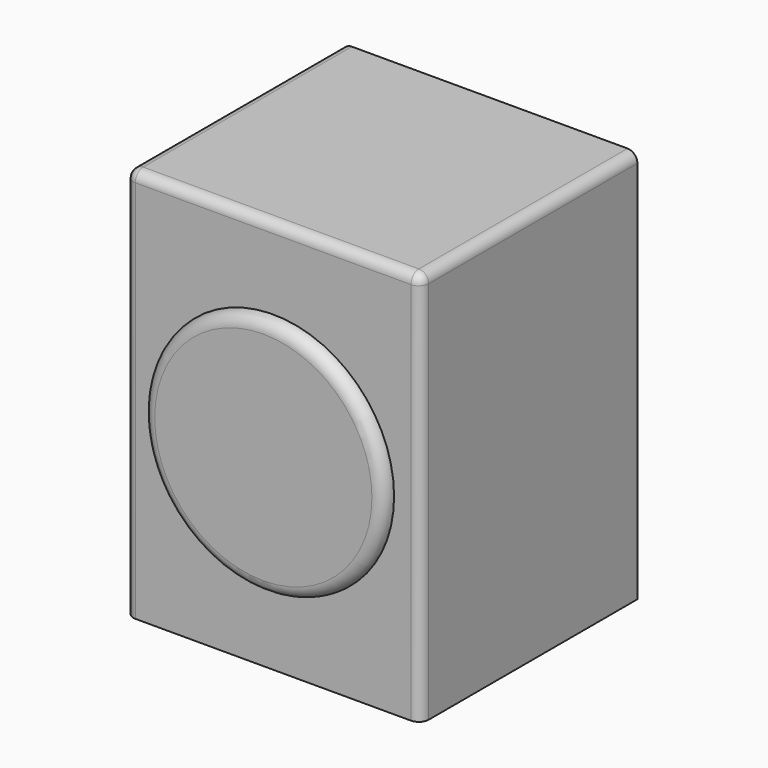
from build123d import *

# Parameters (mm, degrees)
F2_DEPTH = 700
F1_W     = 600
F1_H     = 550
F3_DEPTH = 800
F4_R     = 20
F5_R     = 245.6930164014
F6_DEPTH = 25
F7_R     = 24.99999


# Not quite as in the source:
# - a fillet or chamfer is up to 0.001 mm smaller than in the source, because OpenCascade refuses the exact size


with BuildPart() as f2:
    # F0 (on Top) → F2 (new body)
    with BuildSketch(Plane.XY):
        Polygon((81.1656415462, 504.1027583182), (-518.8343584538, 504.1027583182), (-518.8343584538, -45.8972416818), (-500.8343584538, -45.8972416818), (-500.8343584538, 501.1027583182), (63.1656415462, 501.1027583182), (63.1656415462, -45.8972416818), (81.1656415462, -45.8972416818), align=None)
    extrude(amount=F2_DEPTH)

    # F1 (on Top) → F3 (join)
    with BuildSketch(Plane.XY):
        with Locations((-218.8343584538, 229.1027583182)):
            Rectangle(F1_W, F1_H)
    extrude(amount=F3_DEPTH)

    # F4
    f4_edges = [f2.edges().sort_by_distance(p)[0] for p in [
        (-218.834358, -45.897242, 800),
        (81.165642, 229.102758, 800),
        (-518.834358, 229.102758, 800),
        (81.165642, -45.897242, 400),
        (-518.834358, -45.897242, 400),
    ]]
    fillet(f4_edges, radius=F4_R)

    # F5 (on face) → F6 (join)
    with BuildSketch(Plane.XZ.offset(45.8972416818)):
        with Locations((-218.8343584538, 390)):
            Circle(F5_R)
    extrude(amount=F6_DEPTH)

    # F7 (radius 25 in the source; OpenCascade refuses exactly that, so slightly less here)
    f7_edges = [f2.edges().sort_by_distance(p)[0] for p in [
        (-464.527375, -70.897242, 390),
    ]]
    fillet(f7_edges, radius=F7_R)


solid = f2.part
